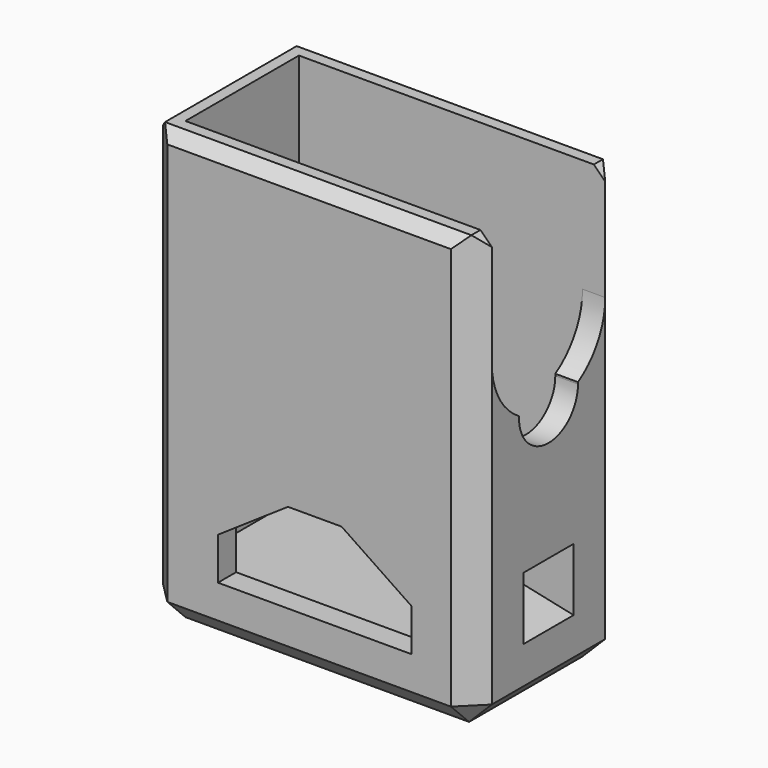
from build123d import *

# Parameters (mm, degrees)
F0_W      = 29
F0_H      = 16.5
F1_DEPTH  = 38.5
F2_T      = -2
F3_DEPTH  = 2.25
F4_SIZE   = 2
F5_SIZE   = 0.99999
F7_DEPTH  = 16.501
F9_DEPTH  = 2
F10_R     = 2
F11_DEPTH = 2.001
F12_W     = 7.54
F12_H     = 7.25
F12_R     = 1.1
F13_DEPTH = 6.35
F14_W     = 5.538
F14_H     = 5.533
F16_W     = 5.538
F16_H     = 4.583


# Not quite as in the source:
# - a fillet or chamfer is up to 0.001 mm smaller than in the source, because OpenCascade refuses the exact size


with BuildPart() as f1:
    # F0 (on Top) → F1 (new body)
    with BuildSketch(Plane.XY):
        with Locations((14.5, 8.25)):
            Rectangle(F0_W, F0_H)
    extrude(amount=F1_DEPTH)

    # F2
    f2_openings = [f1.faces().sort_by_distance(p)[0] for p in [
        (14.5, 8.25, 38.5),
    ]]
    offset(amount=F2_T, openings=f2_openings)

    # F3 (add): a face of the model
    f3_faces = [f1.faces().sort_by_distance(p)[0] for p in [
        (14.5, 8.25, 2),
    ]]
    extrude(f3_faces, amount=F3_DEPTH)

    # F4
    f4_edges = [f1.edges().sort_by_distance(p)[0] for p in [
        (0, 16.5, 19.25),
        (0, 0, 19.25),
        (29, 16.5, 19.25),
        (29, 0, 19.25),
        (14.5, 16.5, 0),
        (14.5, 0, 0),
        (29, 8.25, 0),
        (0, 8.25, 0),
    ]]
    chamfer(f4_edges, length=F4_SIZE)

    # F5 (size 1 in the source; OpenCascade refuses exactly that, so slightly less here)
    f5_edges = [f1.edges().sort_by_distance(p)[0] for p in [
        (14.5, 16.5, 38.5),
        (14.5, 0, 38.5),
        (0, 8.25, 38.5),
        (29, 8.25, 38.5),
    ]]
    chamfer(f5_edges, length=F5_SIZE)

    # F6 (on face) → F7 (cut, through all)
    with BuildSketch(Plane.XZ):
        Polygon((6.464, 8.664), (6.464, 4.94), (23.536, 4.94), (23.536, 8.664), (17.364, 12.834), (12.635, 12.834), align=None)
    extrude(amount=-F7_DEPTH, mode=Mode.SUBTRACT)

    # F8 (on face) → F9 (cut, through all)
    with BuildSketch(Plane.YZ.offset(29)):
        with BuildLine():
            Line((14.5, 38.5), (2, 38.5))
            Line((2, 38.5), (2, 28.5))
            ThreePointArc((2, 28.5), (8.25, 34.75), (14.5, 28.5))
            Line((14.5, 28.5), (14.5, 38.5))
        make_face()
        with BuildLine():
            ThreePointArc((14.5, 28.5), (8.25, 34.75), (2, 28.5))
            Line((2, 28.5), (14.5, 28.5))
        make_face()
        with BuildLine():
            Line((14.5, 28.5), (2, 28.5))
            ThreePointArc((2, 28.5), (2.8024937382, 25.4361502113), (5.0038961688, 23.1590909091))
            ThreePointArc((5.0038961688, 23.1590909091), (8.25, 26.25), (11.4961038312, 23.1590909091))
            ThreePointArc((11.4961038312, 23.1590909091), (13.6975062618, 25.4361502113), (14.5, 28.5))
        make_face()
        with BuildLine():
            ThreePointArc((11.4961038312, 23.1590909091), (8.25, 26.25), (5.0038961688, 23.1590909091))
            ThreePointArc((5.0038961688, 23.1590909091), (8.25, 22.25), (11.4961038312, 23.1590909091))
        make_face()
        with BuildLine():
            ThreePointArc((11.4961038312, 23.1590909091), (8.25, 22.25), (5.0038961688, 23.1590909091))
            ThreePointArc((5.0038961688, 23.1590909091), (8.1704306945, 19.7509741882), (11.5, 23))
            ThreePointArc((11.5, 23), (11.4990258118, 23.0795693055), (11.4961038312, 23.1590909091))
        make_face()
    extrude(amount=-F9_DEPTH, mode=Mode.SUBTRACT)

    # F10 (on face) → F11 (cut, through all)
    with BuildSketch(Plane.YZ.offset(2)):
        with Locations((8.25, 23)):
            Circle(F10_R)
    extrude(amount=-F11_DEPTH, mode=Mode.SUBTRACT)

    # F12 (on face) → F13 (join)
    with BuildSketch(Plane.YZ.offset(29)):
        with Locations((8.25, 7.875)):
            Rectangle(F12_W, F12_H)
        with Locations((8.25, 9)):
            Circle(F12_R, mode=Mode.SUBTRACT)
    extrude(amount=-F13_DEPTH)

    # F14 (on face) → F17 section 0
    with BuildSketch(Plane.YZ.offset(29)):
        with Locations((8.25, 8.0385)):
            Rectangle(F14_W, F14_H)
    # F16 (on offset) → F17 section 1
    with BuildSketch(Plane.YZ.offset(24.55)):
        with Locations((8.25, 8.5135)):
            Rectangle(F16_W, F16_H)
    loft(mode=Mode.SUBTRACT)


solid = f1.part
